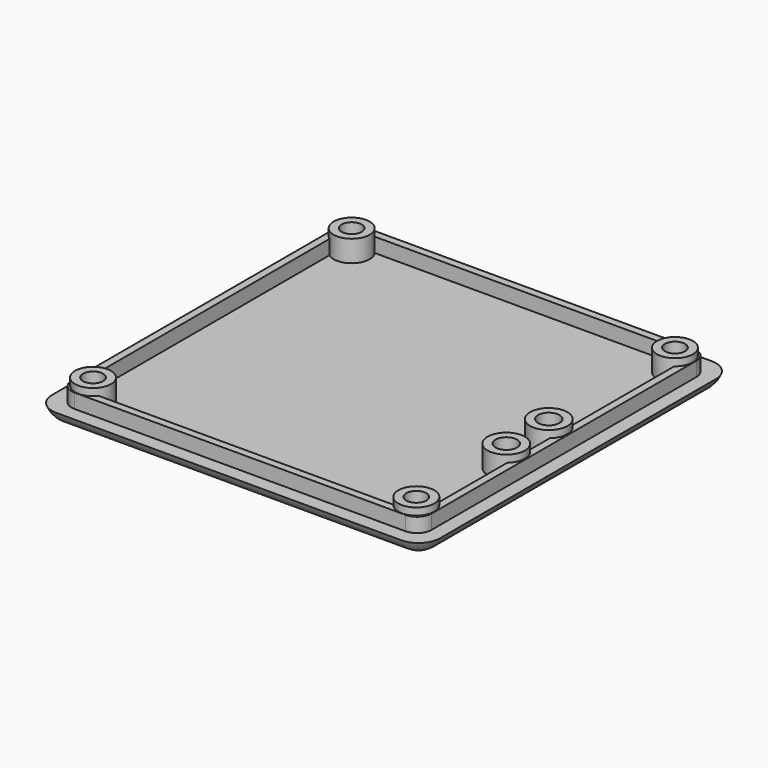
from build123d import *

# Parameters (mm, degrees)
F0_W         = 54
F0_H         = 54
F1_DEPTH     = 2
F2_R         = 3
F3_T1_DEPTH  = 48
F3_T3_DEPTH  = 48
F3_T6_ANGLE  = 90
F3_T8_ANGLE  = 90
F3_T10_ANGLE = 90
F3_T12_ANGLE = 90
F4_W         = 50.1
F4_H         = 50.1
F4_W_2       = 48
F4_H_2       = 48
F5_DEPTH     = 2
F6_R         = 2.5
F6_R_2       = 1.4
F7_DEPTH     = 3
F8_R         = 2
F9_R         = 2.6
F9_R_2       = 1.5
F10_DEPTH    = 3
F11_R        = 1.5
F12_DEPTH    = 25


# Not quite as in the source:
# - a fillet or chamfer that OpenCascade refuses, or shapes differently, is made with other operations: its cross-section is extruded or revolved along the edge and cut away or added


with BuildPart() as f1:
    # F0 (on Top) → F1 (new body)
    with BuildSketch(Plane.XY):
        Rectangle(F0_W, F0_H)
    extrude(amount=F1_DEPTH)

    # F2
    f2_edges = [f1.edges().sort_by_distance(p)[0] for p in [
        (-27, -27, 1),
        (-27, 27, 1),
        (27, 27, 1),
        (27, -27, 1),
    ]]
    fillet(f2_edges, radius=F2_R)

    # F3: fillet of radius 3 on 8 edges, made by hand

    # F3_s2 → F3_t1 (cut)
    with BuildSketch(Plane.YZ.offset(-24)):
        with BuildLine():
            ThreePointArc((27, 2), (25.9036236828, 0.5505102572), (24.1715728753, 0))
            Line((24.1715728753, 0), (27, 0))
            Line((27, 0), (27, 2))
        make_face()
        with BuildLine():
            ThreePointArc((-24.1715728753, 0), (-25.9036236828, 0.5505102572), (-27, 2))
            Line((-27, 2), (-27, 0))
            Line((-27, 0), (-24.1715728753, 0))
        make_face()
    extrude(amount=F3_T1_DEPTH, mode=Mode.SUBTRACT)

    # F3_s4 → F3_t3 (cut)
    with BuildSketch(Plane.XZ.offset(-24)):
        with BuildLine():
            ThreePointArc((24.1715728753, 0), (25.9036236828, 0.5505102572), (27, 2))
            Line((27, 2), (27, 0))
            Line((27, 0), (24.1715728753, 0))
        make_face()
        with BuildLine():
            ThreePointArc((-24.1715728753, 0), (-25.9036236828, 0.5505102572), (-27, 2))
            Line((-27, 2), (-27, 0))
            Line((-27, 0), (-24.1715728753, 0))
        make_face()
    extrude(amount=F3_T3_DEPTH, mode=Mode.SUBTRACT)

    # F3_s5 → F3_t6 (revolve, cut)
    with BuildSketch(Plane.YZ.offset(24)):
        with BuildLine():
            ThreePointArc((24.1715728753, 0), (25.9036236828, 0.5505102572), (27, 2))
            Line((27, 2), (27, 0))
            Line((27, 0), (24.1715728753, 0))
        make_face()
    revolve(axis=Axis((24, 24, 0), (0, 0, -1)), revolution_arc=F3_T6_ANGLE, mode=Mode.SUBTRACT)

    # F3_s7 → F3_t8 (revolve, cut)
    with BuildSketch(Plane.YZ.offset(-24)):
        with BuildLine():
            ThreePointArc((24.1715728753, 0), (25.9036236828, 0.5505102572), (27, 2))
            Line((27, 2), (27, 0))
            Line((27, 0), (24.1715728753, 0))
        make_face()
    revolve(axis=Axis((-24, 24, 0), (0, 0, 1)), revolution_arc=F3_T8_ANGLE, mode=Mode.SUBTRACT)

    # F3_s9 → F3_t10 (revolve, cut)
    with BuildSketch(Plane.YZ.offset(24)):
        with BuildLine():
            ThreePointArc((-24.1715728753, 0), (-25.9036236828, 0.5505102572), (-27, 2))
            Line((-27, 2), (-27, 0))
            Line((-27, 0), (-24.1715728753, 0))
        make_face()
    revolve(axis=Axis((24, -24, 0), (0, 0, 1)), revolution_arc=F3_T10_ANGLE, mode=Mode.SUBTRACT)

    # F3_s11 → F3_t12 (revolve, cut)
    with BuildSketch(Plane.XZ.offset(24)):
        with BuildLine():
            ThreePointArc((-24.1715728753, 0), (-25.9036236828, 0.5505102572), (-27, 2))
            Line((-27, 2), (-27, 0))
            Line((-27, 0), (-24.1715728753, 0))
        make_face()
    revolve(axis=Axis((-24, -24, 0), (0, 0, 1)), revolution_arc=F3_T12_ANGLE, mode=Mode.SUBTRACT)

    # F4 (on face) → F5 (join)
    with BuildSketch(Plane.XY.offset(2)):
        Rectangle(F4_W, F4_H)
        Rectangle(F4_W_2, F4_H_2, mode=Mode.SUBTRACT)
    extrude(amount=F5_DEPTH)

    # F6 (on face) → F7 (join)
    with BuildSketch(Plane.XY.offset(2)):
        with Locations((-22.5, 22.5)):
            Circle(F6_R)
        with Locations((-22.5, 22.5)):
            Circle(F6_R_2, mode=Mode.SUBTRACT)
        with Locations((22.5, 22.5)):
            Circle(F6_R)
        with Locations((22.5, 22.5)):
            Circle(F6_R_2, mode=Mode.SUBTRACT)
        with Locations((22.5, -22.5)):
            Circle(F6_R)
        with Locations((22.5, -22.5)):
            Circle(F6_R_2, mode=Mode.SUBTRACT)
        with Locations((-22.5, -22.5)):
            Circle(F6_R)
        with Locations((-22.5, -22.5)):
            Circle(F6_R_2, mode=Mode.SUBTRACT)
    extrude(amount=F7_DEPTH)

    # F8
    f8_edges = [f1.edges().sort_by_distance(p)[0] for p in [
        (-25.05, -25.05, 3),
        (25.05, -25.05, 3),
        (25.05, 25.05, 3),
        (-25.05, 25.05, 3),
    ]]
    fillet(f8_edges, radius=F8_R)

    # F9 (on face) → F10 (join)
    with BuildSketch(Plane.XY.offset(2)):
        with Locations((22.3, 0.8)):
            Circle(F9_R)
        with Locations((22.3, 0.8)):
            Circle(F9_R_2, mode=Mode.SUBTRACT)
        with Locations((22.3, -6.6)):
            Circle(F9_R)
        with Locations((22.3, -6.6)):
            Circle(F9_R_2, mode=Mode.SUBTRACT)
    extrude(amount=F10_DEPTH)

    # F11 (on face) → F12 (cut)
    with BuildSketch(Plane.XY.offset(2)):
        with Locations((22.3, 0.8)):
            Circle(F11_R)
        with Locations((22.3, -6.6)):
            Circle(F11_R)
    extrude(amount=-F12_DEPTH, mode=Mode.SUBTRACT)


solid = f1.part
